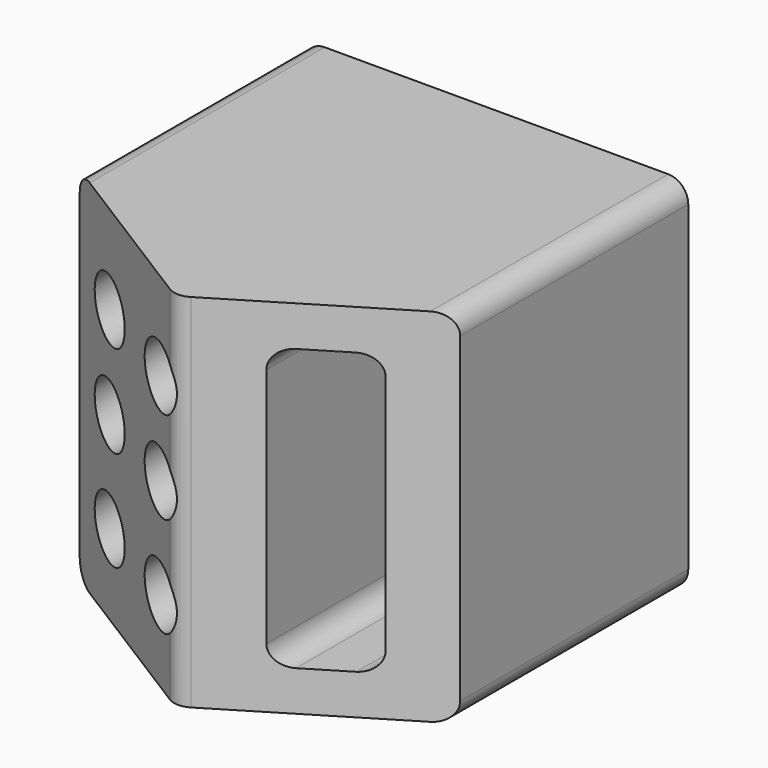
from build123d import *

# Parameters (mm, degrees)
F0_W        = 95.5598546359
F0_H        = 90
F1_DEPTH    = 100
F2_R        = 5
F3_W        = 20
F3_H        = 70
F3_R        = 7.5
F4_DEPTH    = 80
F5_T1_DEPTH = 92.4997500025
F7_DEPTH    = 90
F8_T1_DEPTH = 105.435292613


# Not quite as in the source:
# - a fillet or chamfer that OpenCascade refuses, or shapes differently, is made with other operations: its cross-section is extruded or revolved along the edge and cut away or added


with BuildPart() as f1:
    # F0 (on Front) → F1 (new body)
    with BuildSketch(Plane.XZ):
        with Locations((47.7799273179, 45)):
            Rectangle(F0_W, F0_H)
    extrude(amount=F1_DEPTH)

    # F2
    f2_edges = [f1.edges().sort_by_distance(p)[0] for p in [
        (95.559855, -50, 90),
        (95.559855, -50, 0),
        (0, -50, 0),
        (0, -50, 90),
    ]]
    fillet(f2_edges, radius=F2_R)

    # F3 (on face) → F4 (cut)
    with BuildSketch(Plane.XZ.offset(100)):
        with Locations((73.0598546359, 45)):
            Rectangle(F3_W, F3_H)
        with Locations((15, 45)):
            Circle(F3_R)
        with Locations((15, 68)):
            Circle(F3_R)
        with Locations((40, 45)):
            Circle(F3_R)
        with Locations((40, 68)):
            Circle(F3_R)
        with Locations((15, 20)):
            Circle(F3_R)
        with Locations((40, 20)):
            Circle(F3_R)
    extrude(amount=-F4_DEPTH, mode=Mode.SUBTRACT)

    # F5: fillet of radius 5 on 4 edges, made by hand

    # F5_s2 → F5_t1 (join)
    with BuildSketch(Plane.XZ.offset(7.5002499975)):
        with BuildLine():
            ThreePointArc((68.0597546359, 80.0001), (64.5242207299, 78.5356339059), (63.0597546359, 75.0001))
            Line((63.0597546359, 75.0001), (62.9597546359, 75.0001))
            ThreePointArc((62.9597546359, 75.0001), (62.9598546359, 77.50005), (62.9598546359, 80))
            Line((62.9598546359, 80), (63.0598546359, 80.1))
            ThreePointArc((63.0598546359, 80.1), (65.5598046359, 80.1), (68.0597546359, 80.1001))
            Line((68.0597546359, 80.1001), (68.0597546359, 80.0001))
        make_face()
        with BuildLine():
            ThreePointArc((78.0599546359, 80.0001), (81.5954885418, 78.5356339059), (83.0599546359, 75.0001))
            Line((83.0599546359, 75.0001), (83.1599546359, 75.0001))
            ThreePointArc((83.1599546359, 75.0001), (83.1598546359, 77.50005), (83.1598546359, 80))
            Line((83.1598546359, 80), (83.0598546359, 80.1))
            ThreePointArc((83.0598546359, 80.1), (80.5599046359, 80.1), (78.0599546359, 80.1001))
            Line((78.0599546359, 80.1001), (78.0599546359, 80.0001))
        make_face()
        with BuildLine():
            ThreePointArc((78.0599546359, 9.9999), (81.5954885418, 11.4643660941), (83.0599546359, 14.9999))
            Line((83.0599546359, 14.9999), (83.1599546359, 14.9999))
            ThreePointArc((83.1599546359, 14.9999), (83.1598546359, 12.49995), (83.1598546359, 10))
            Line((83.1598546359, 10), (83.0598546359, 9.9))
            ThreePointArc((83.0598546359, 9.9), (80.5599046359, 9.9), (78.0599546359, 9.8999))
            Line((78.0599546359, 9.8999), (78.0599546359, 9.9999))
        make_face()
        with BuildLine():
            ThreePointArc((63.0597546359, 14.9999), (64.5242207299, 11.4643660941), (68.0597546359, 9.9999))
            Line((68.0597546359, 9.9999), (68.0597546359, 9.8999))
            ThreePointArc((68.0597546359, 9.8999), (65.5598046359, 9.9), (63.0598546359, 9.9))
            Line((63.0598546359, 9.9), (62.9598546359, 10))
            ThreePointArc((62.9598546359, 10), (62.9598546359, 12.49995), (62.9597546359, 14.9999))
            Line((62.9597546359, 14.9999), (63.0597546359, 14.9999))
        make_face()
    extrude(amount=F5_T1_DEPTH)

    # F6 (on face) → F7 (cut)
    with BuildSketch(Plane(origin=(0, 0, 0), x_dir=(1, 0, 0), z_dir=(0, 0, -1))):
        Polygon((0, 124.7042194009), (0, 70), (47.7799273179, 100), (97.1999242902, 70), (97.1999242902, 124.7042194009), align=None)
    extrude(amount=-F7_DEPTH, mode=Mode.SUBTRACT)

    # F8: fillet of radius 5 on 1 edges, made by hand

    # F8_s2 → F8_t1 (cut)
    with BuildSketch(Plane.XY.offset(-7.7176463065)):
        with BuildLine():
            ThreePointArc((45.1654951007, -98.3584536244), (47.7865363785, -99.1238075774), (50.4188247907, -98.3980791373))
            Line((50.4188247907, -98.3980791373), (47.7799273179, -100))
            Line((47.7799273179, -100), (45.1654951007, -98.3584536244))
        make_face()
    extrude(amount=F8_T1_DEPTH, mode=Mode.SUBTRACT)


solid = f1.part
